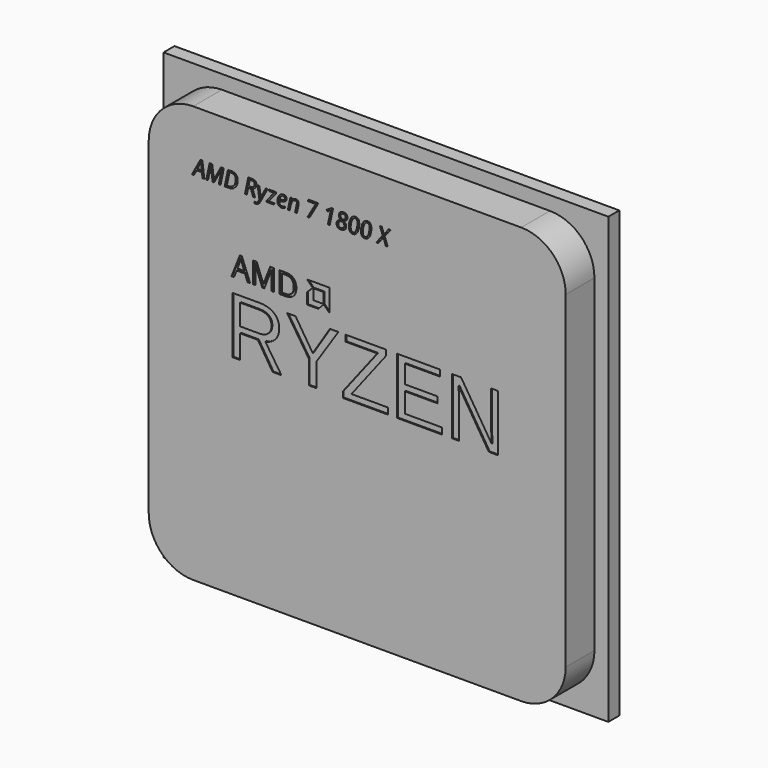
from build123d import *

# Parameters (mm, degrees)
F0_W           = 40
F0_H           = 40
F1_DEPTH       = 1.23
F3_DEPTH       = 3.23
F4_W           = 0.8763410151
F4_H           = 0.9456500411
F4_TEXT_SIZE   = 1.9735827723
F4_TEXT_SIZE_2 = 2.6449924232
F4_TEXT_SIZE_3 = 7.4029519271
F5_DEPTH       = 0.1


# Not quite as in the source:
# - Text() gives the source's letters only with a copy of the font that has no kerning and outlines rounded to 1/6400 em; it was checked with that copy


with BuildPart() as f1:
    # F0 (on Front) → F1 (new body)
    with BuildSketch(Plane.XZ):
        with Locations((20, 20)):
            Rectangle(F0_W, F0_H)
    extrude(amount=F1_DEPTH)

    # F2 (on face) → F3 (join)
    with BuildSketch(Plane.XZ.offset(1.23)):
        with BuildLine():
            Line((34.75, 38.75), (5.25, 38.75))
            ThreePointArc((5.25, 38.75), (2.4215728753, 37.5784271247), (1.25, 34.75))
            Line((1.25, 34.75), (1.25, 5.25))
            ThreePointArc((1.25, 5.25), (2.4215728753, 2.4215728753), (5.25, 1.25))
            Line((5.25, 1.25), (34.75, 1.25))
            ThreePointArc((34.75, 1.25), (37.5784271247, 2.4215728753), (38.75, 5.25))
            Line((38.75, 5.25), (38.75, 34.75))
            ThreePointArc((38.75, 34.75), (37.5784271247, 37.5784271247), (34.75, 38.75))
        make_face()
    extrude(amount=F3_DEPTH)

    # F4 (on face) → F5 (cut)
    with BuildSketch(Plane.XZ.offset(4.46)):
        Polygon((17.4968975112, 28.3782516122), (15.4968975112, 28.3782516122), (15.9968975112, 27.8782516122), (15.4968975112, 27.3782516122), (15.4968975112, 26.3782516122), (16.4968975112, 26.3782516122), (16.9968975112, 26.8782516122), (17.4968975112, 26.3782516122), align=None)
        with Locations((16.5237821639, 27.386829257)):
            Rectangle(F4_W, F4_H, mode=Mode.SUBTRACT)
        with Locations((5.25, 33.329020404)):
            Text('AMD Ryzen 7 1800 X', F4_TEXT_SIZE, font='Open Sans', font_style=FontStyle.ITALIC, text_align=(TextAlign.LEFT, TextAlign.BOTTOM))
        with Locations((8.696271832, 26.4156680152)):
            Text('AMD', F4_TEXT_SIZE_2, font='Open Sans', text_align=(TextAlign.LEFT, TextAlign.BOTTOM))
        with Locations((8.1822493368, 20.037875014)):
            Text('RYZEN', F4_TEXT_SIZE_3, font='Arimo', text_align=(TextAlign.LEFT, TextAlign.BOTTOM))
    extrude(amount=-F5_DEPTH, mode=Mode.SUBTRACT)


solid = f1.part
